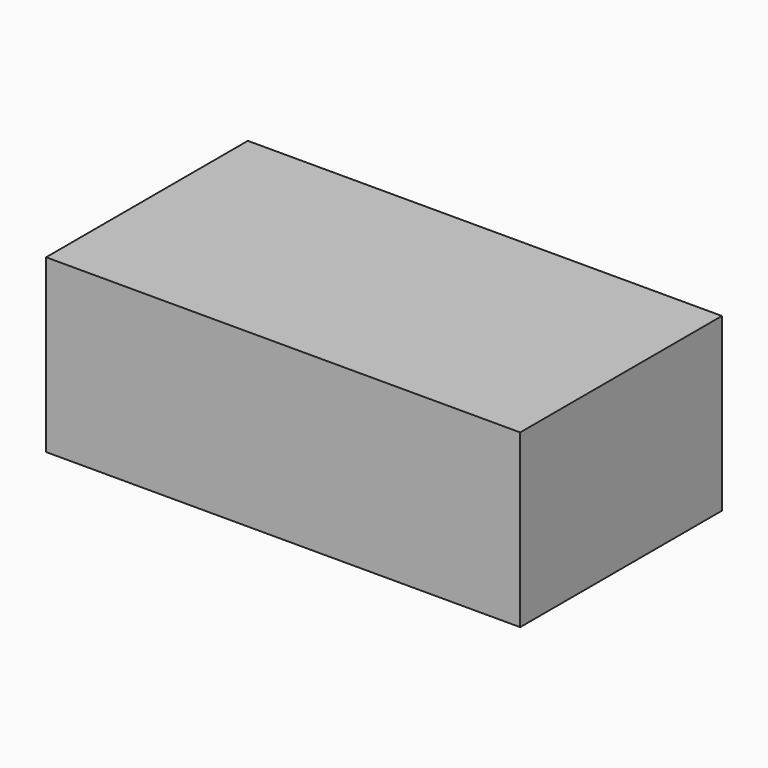
from build123d import *

# Parameters (mm, degrees)
F2_W     = 1193.8
F2_H     = 431.8
F3_DEPTH = 635
F6_DEPTH = 12.7
F7_DEPTH = 12.7
F5_W     = 355.6
F5_H     = 12.7
F8_DEPTH = 12.7
F9_DEPTH = 12.7


# Not quite as in the source:
# - a variable given as a bare number and used for a length is read in inches; the dataset says mm whatever the document's units were


with BuildPart() as f3:
    # F2 (on Front) → F3 (new body)
    with BuildSketch(Plane.XZ):
        with Locations((596.9, 215.9)):
            Rectangle(F2_W, F2_H)
    extrude(amount=F3_DEPTH)


with BuildPart() as f6:
    # F5 (on offset) → F6 (new body)
    with BuildSketch(Plane(origin=(152.4, 0, 0), x_dir=(0, -1, 0), z_dir=(-1, 0, 0))):
        Polygon((76.2, 387.35), (127, 387.35), (139.7, 387.35), (495.3, 387.35), (508, 387.35), (558.8, 387.35), (558.8, 400.05), (76.2, 400.05), align=None)
    extrude(amount=-F6_DEPTH)


with BuildPart() as f7:
    # F5 (on offset) → F7 (new body)
    with BuildSketch(Plane(origin=(152.4, 0, 0), x_dir=(0, -1, 0), z_dir=(-1, 0, 0))):
        Polygon((127, 387.35), (127, 0), (139.7, 0), (139.7, 152.4), (139.7, 165.1), (139.7, 387.35), align=None)
    extrude(amount=-F7_DEPTH)


with BuildPart() as f8:
    # F5 (on offset) → F8 (new body)
    with BuildSketch(Plane(origin=(152.4, 0, 0), x_dir=(0, -1, 0), z_dir=(-1, 0, 0))):
        with Locations((317.5, 158.75)):
            Rectangle(F5_W, F5_H)
    extrude(amount=-F8_DEPTH)


with BuildPart() as f9:
    # F5 (on offset) → F9 (new body)
    with BuildSketch(Plane(origin=(152.4, 0, 0), x_dir=(0, -1, 0), z_dir=(-1, 0, 0))):
        Polygon((495.3, 165.1), (495.3, 152.4), (495.3, 0), (508, 0), (508, 387.35), (495.3, 387.35), align=None)
    extrude(amount=-F9_DEPTH)


solid = Compound([f3.part, f6.part, f7.part, f8.part, f9.part])
